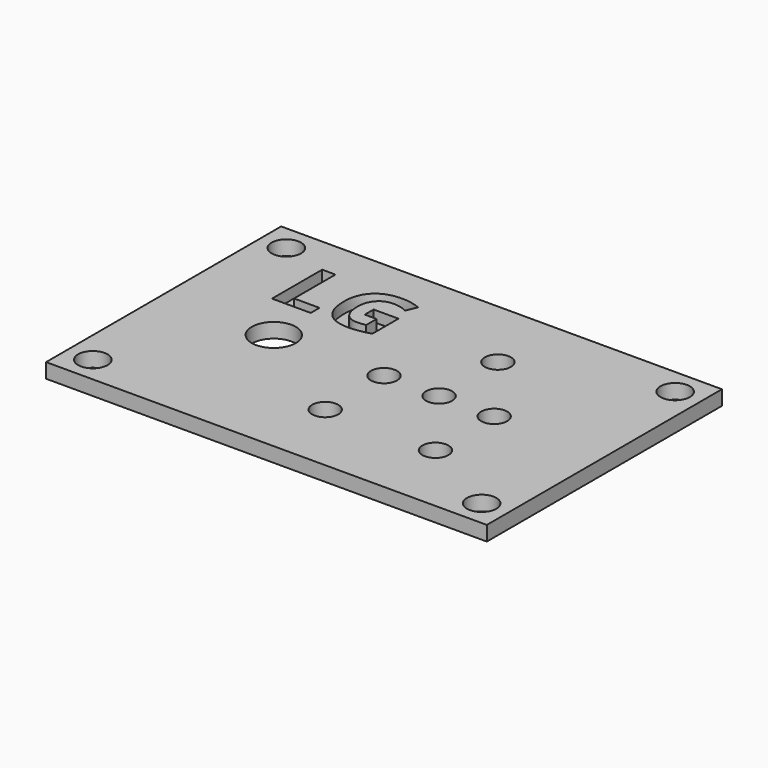
from build123d import *

# Parameters (mm, degrees)
F0_W         = 60
F0_H         = 40
F0_R         = 2
F0_R_2       = 1.775
F0_R_3       = 3
F1_DEPTH     = 2
F2_TEXT_SIZE = 11.9568902947
F3_DEPTH     = 1.5


# Not quite as in the source:
# - Text() gives the source's letters only with a copy of the font that has no kerning and outlines rounded to 1/6400 em; it was checked with that copy


with BuildPart() as f1:
    # F0 (on Top) → F1 (new body)
    with BuildSketch(Plane.XY):
        Rectangle(F0_W, F0_H)
        with Locations((-26.4644660941, -16.4644660941)):
            Circle(F0_R, mode=Mode.SUBTRACT)
        with Locations((26.4644660941, -16.4644660941)):
            Circle(F0_R, mode=Mode.SUBTRACT)
        with Locations((0, -10)):
            Circle(F0_R_2, mode=Mode.SUBTRACT)
        with Locations((15, -10)):
            Circle(F0_R_2, mode=Mode.SUBTRACT)
        with Locations((-15, 0)):
            Circle(F0_R_3, mode=Mode.SUBTRACT)
        with Locations((-26.4644660941, 16.4644660941)):
            Circle(F0_R, mode=Mode.SUBTRACT)
        Circle(F0_R_2, mode=Mode.SUBTRACT)
        with Locations((7.5, 0)):
            Circle(F0_R_2, mode=Mode.SUBTRACT)
        with Locations((15, 0)):
            Circle(F0_R_2, mode=Mode.SUBTRACT)
        with Locations((7.5, 10)):
            Circle(F0_R_2, mode=Mode.SUBTRACT)
        with Locations((26.4644660941, 16.4644660941)):
            Circle(F0_R, mode=Mode.SUBTRACT)
    extrude(amount=-F1_DEPTH)

    # F2 (on face) → F3 (cut)
    with BuildSketch(Plane.XY):
        with Locations((-21.4497018605, 6.4105778001)):
            Text('LG', F2_TEXT_SIZE, font='Open Sans', font_style=FontStyle.BOLD, text_align=(TextAlign.LEFT, TextAlign.BOTTOM))
    extrude(amount=-F3_DEPTH, mode=Mode.SUBTRACT)


solid = f1.part
